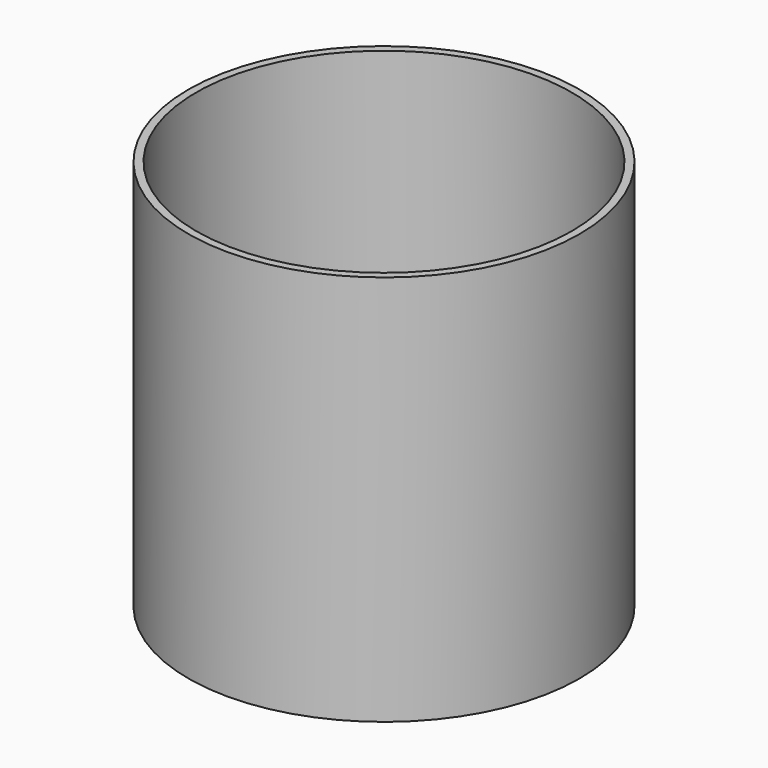
from build123d import *

# Parameters (mm, degrees)
F0_R          = 63.5
F1_DEPTH      = 63.5
F1_DEPTH_BACK = 63.5
F2_T          = -2.54


# Not quite as in the source:
# - the program builds the solid bodies; features that only make, move or delete a surface that nothing else refers to are left out


with BuildPart() as f1:
    # F0 (on Top) → F1 (new body, two sides)
    with BuildSketch(Plane.XY) as f1_sk:
        Circle(F0_R)
    extrude(amount=F1_DEPTH)
    extrude(f1_sk.sketch, amount=-F1_DEPTH_BACK)

    # F2
    f2_openings = [f1.faces().sort_by_distance(p)[0] for p in [
        (0, 0, 63.5),
    ]]
    offset(amount=F2_T, openings=f2_openings)


solid = f1.part
